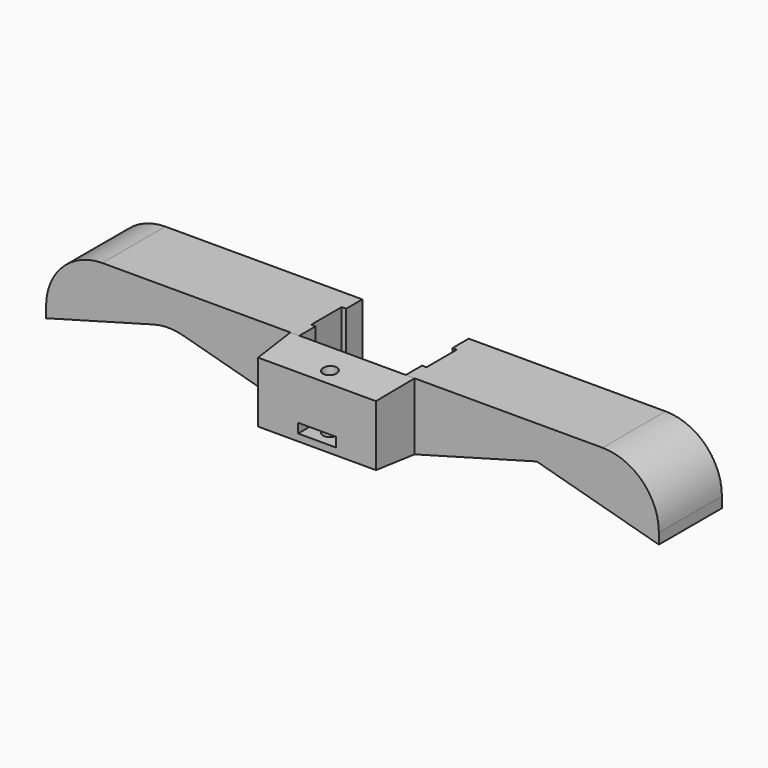
from build123d import *

# Parameters (mm, degrees)
F0_W     = 14
F0_H     = 15.1035089948
F1_DEPTH = 17.78
F2_W     = 28
F2_H     = 15.1035089948
F3_DEPTH = 10
F3_TAPER = 4
F4_R     = 12.7
F5_W     = 1
F5_H     = 8.6030326784
F5_W_2   = 24
F5_H_2   = 4.5689390972
F5_R     = 1.5875
F6_DEPTH = 15.1045090948
F7_W     = 8.5285408422
F7_H     = 2.1393047646
F8_DEPTH = 7.62


# Not quite as in the source:
# - a feature names something its author has since deleted; it is built from what else it names


with BuildPart() as f1:
    # F0 (on Front) → F1 (new body)
    with BuildSketch(Plane.XZ):
        Polygon((-16, 0.5480427082), (-14, 0), (-14, 15.1035089948), (-16, 15.1035089948), align=None)
        with BuildLine():
            Line((-41.559, 7.5517544974), (-16, 0.5480427082))
            Line((-16, 0.5480427082), (-16, 15.1035089948))
            Line((-16, 15.1035089948), (-56.418, 15.1035089948))
            ThreePointArc((-56.418, 15.1035089948), (-65.3982561211, 11.3837651159), (-69.118, 2.4035089948))
            Line((-69.118, 2.4035089948), (-69.118, 0))
            Line((-69.118, 0), (-41.559, 7.5517544974))
        make_face()
        with Locations((-7, 7.5517544974)):
            Rectangle(F0_W, F0_H)
        with Locations((7, 7.5517544974)):
            Rectangle(F0_W, F0_H)
        with BuildLine():
            Line((16, 15.1035089948), (16, 0.5480427082))
            Line((16, 0.5480427082), (41.559, 7.5517544974))
            Line((41.559, 7.5517544974), (69.118, 0))
            Line((69.118, 0), (69.118, 2.4035089948))
            ThreePointArc((69.118, 2.4035089948), (65.3982561211, 11.3837651159), (56.418, 15.1035089948))
            Line((56.418, 15.1035089948), (16, 15.1035089948))
        make_face()
        Polygon((14, 15.1035089948), (14, 0), (16, 0.5480427082), (16, 15.1035089948), align=None)
    extrude(amount=F1_DEPTH)

    # F2 (on face) → F3 (join)
    with BuildSketch(Plane.XZ.offset(17.78)):
        with Locations((0, 7.5517544974)):
            Rectangle(F2_W, F2_H)
    extrude(amount=F3_DEPTH, taper=F3_TAPER)

    # F4
    f4_edges = [f1.edges().sort_by_distance(p)[0] for p in [
        (-41.559, -8.89, 7.551754),
    ]]
    fillet(f4_edges, radius=F4_R)

    # F5 (on face) → F6 (cut, through all)
    with BuildSketch(Plane(origin=(0, 0, 0), x_dir=(1, 0, 0), z_dir=(0, 0, -1))):
        with Locations((-12.5, 8.8704554364)):
            Rectangle(F5_W, F5_H)
        with Locations((0, 8.8704554364)):
            Rectangle(F5_W_2, F5_H)
        with Locations((0, 2.2844695486)):
            Rectangle(F5_W_2, F5_H_2)
        with Locations((12.5, 8.8704554364)):
            Rectangle(F5_W, F5_H)
        with Locations((0, 15.4564413242)):
            Rectangle(F5_W_2, F5_H_2)
        with Locations((0, 24.13)):
            Circle(F5_R)
    extrude(amount=-F6_DEPTH, mode=Mode.SUBTRACT)

    # F7 (on face) → F8 (cut)
    with BuildSketch(Plane.XZ.offset(27.78)):
        with Locations((0, 3.333498491)):
            Rectangle(F7_W, F7_H)
    extrude(amount=-F8_DEPTH, mode=Mode.SUBTRACT)


solid = f1.part
